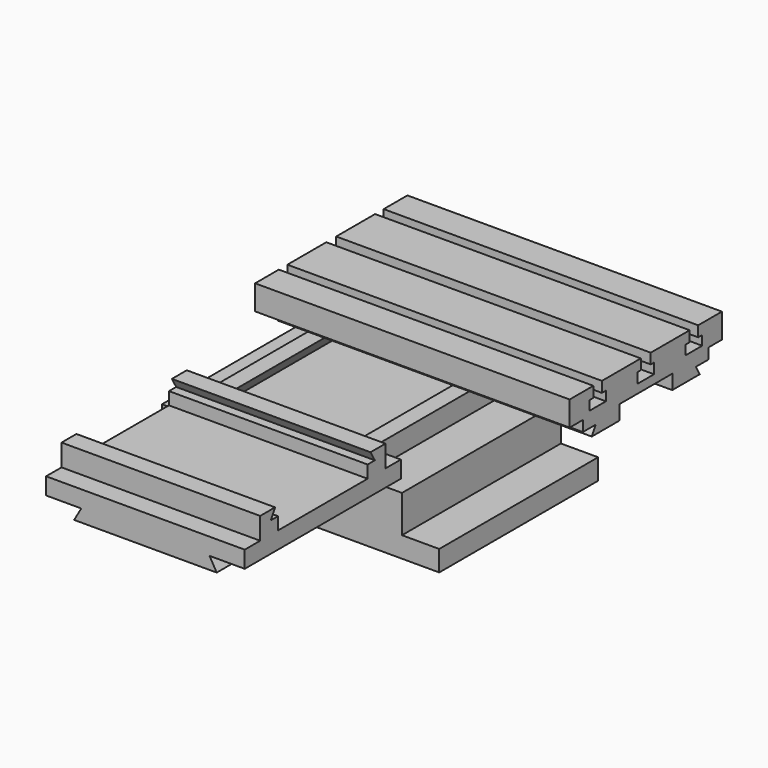
from build123d import *

# Parameters (mm, degrees)
F1_DEPTH = 152.4
F3_DEPTH = 241.3
F5_DEPTH = 152.4
F7_DEPTH = 152.4


with BuildPart() as f1:
    # F0 (on Front) → F1 (new body)
    with BuildSketch(Plane.XZ):
        Polygon((-110.1936613465, -46.4599046108), (-110.1936613465, -62.3349046108), (131.1063386535, -62.3349046108), (131.1063386535, -46.4599046108), (102.5313386535, -46.4599046108), (102.5313386535, -17.8849046108), (70.7813386535, -17.8849046108), (70.7813386535, -2.0099046108), (58.0813386535, -2.0099046108), (63.5805999675, -11.5349046108), (-45.8429226605, -11.5349046108), (-40.3436613465, -2.0099046108), (-53.0436613465, -2.0099046108), (-53.0436613465, -17.8849046108), (-81.6186613465, -17.8849046108), (-81.6186613465, -46.4599046108), align=None)
    extrude(amount=-F1_DEPTH)


with BuildPart() as f3:
    # F2 (on Right) → F3 (new body)
    with BuildSketch(Plane.YZ):
        Polygon((12.3105041872, 68.34122984), (8.5416771, 61.81342984), (34.925, 61.81342984), (34.925, 72.92592984), (85.725, 72.92592984), (85.725, 61.81342984), (112.1083229, 61.81342984), (108.3394958128, 68.34122984), (120.65, 68.34122984), (120.65, 76.52002984), (133.35, 76.52002984), (133.35, 95.49382984), (110.5916, 95.49382984), (110.5916, 87.36582984), (114.427, 87.36582984), (114.427, 80.12682984), (98.552, 80.12682984), (98.552, 87.36582984), (102.3874, 87.36582984), (102.3874, 95.49382984), (65.0875, 95.49382984), (65.0875, 87.55632984), (68.2625, 87.55632984), (68.2625, 79.61882984), (52.3875, 79.61882984), (52.3875, 87.55632984), (55.5625, 87.55632984), (55.5625, 95.49382984), (18.2626, 95.49382984), (18.2626, 87.36582984), (22.098, 87.36582984), (22.098, 80.12682984), (6.223, 80.12682984), (6.223, 87.36582984), (10.0584, 87.36582984), (10.0584, 95.49382984), (-12.7, 95.49382984), (-12.7, 76.52002984), (0, 76.52002984), (0, 68.34122984), align=None)
    extrude(amount=F3_DEPTH)


with BuildPart() as f5:
    # F4 (on Right) → F5 (new body)
    with BuildSketch(Plane.YZ):
        Polygon((-213.1368674653, 46.6388186438), (-213.1368674653, 33.6848186438), (-63.4038674653, 33.6848186438), (-63.4038674653, 46.6388186438), (-78.2120674653, 46.6388186438), (-78.2120674653, 63.4028186438), (-92.4995674653, 63.4028186438), (-88.378787654, 56.2654186438), (-95.3062674653, 56.2654186438), (-95.3062674653, 46.6388186438), (-181.2344674653, 46.6388186438), (-181.2344674653, 56.2654186438), (-188.1619472766, 56.2654186438), (-184.0411674653, 63.4028186438), (-198.3286674653, 63.4028186438), (-198.3286674653, 46.6388186438), align=None)
    extrude(amount=F5_DEPTH)

    # F6 (on face) → F7 (join)
    with BuildSketch(Plane.XZ.offset(213.1368674653)):
        Polygon((125.4125, 33.6848186438), (26.9875, 33.6848186438), (21.4884, 24.1600980479), (130.9116, 24.1600980479), align=None)
    extrude(amount=-F7_DEPTH)


solid = Compound([f1.part, f3.part, f5.part])
